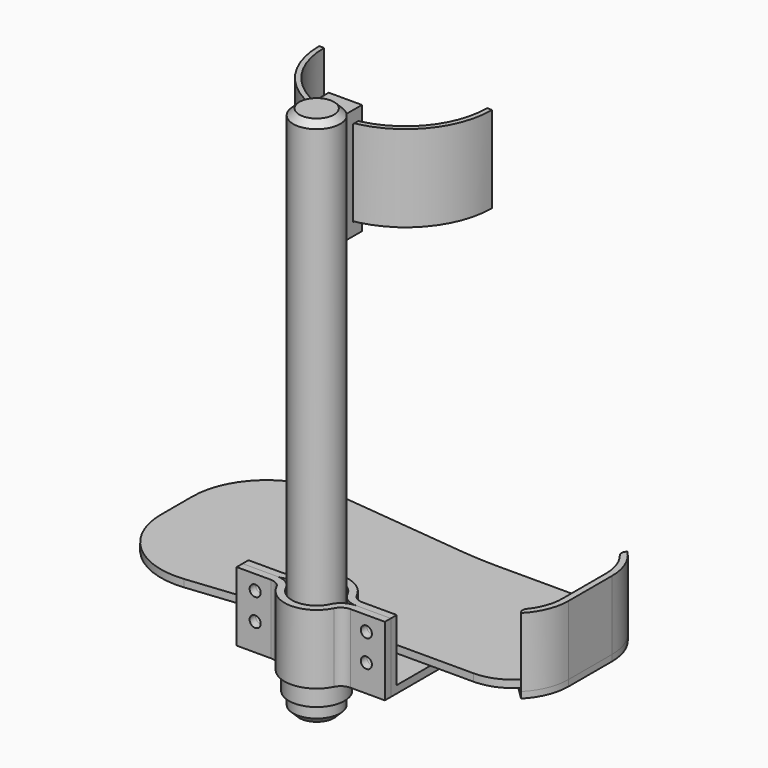
from build123d import *

# Parameters (mm, degrees)
F1_DEPTH  = 6
F2_R      = 60
F3_R      = 40
F4_R      = 300
F5_R      = 10
F6_DEPTH  = 6
F8_DEPTH  = 6
F9_DEPTH  = 50
F10_R     = 5
F12_DEPTH = 5
F14_DEPTH = 6
F16_DEPTH = 50
F17_R     = 10
F18_R     = 15
F20_DEPTH = 56
F21_R     = 4.5
F22_DEPTH = 25
F23_R     = 4.5
F24_DEPTH = 25
F25_R     = 19
F26_DEPTH = 400
F27_DEPTH = 30
F28_SIZE  = 5
F29_R     = 22.5
F29_R_2   = 19
F30_DEPTH = 15
F31_SIZE  = 5
F34_DEPTH = 90
F36_W     = 26.8700576851
F36_H     = 4
F37_DEPTH = 70
F39_DEPTH = 70


with BuildPart() as f1:
    # F0 (on Top) → F1 (new body)
    with BuildSketch(Plane.XY):
        Polygon((20, 62.0046741232), (-175, 82.5), (-175, -82.5), (20, -62.0046741232), (155, -62.0046741232), (155, 62.0046741232), align=None)
    extrude(amount=F1_DEPTH)

    # F2
    f2_edges = [f1.edges().sort_by_distance(p)[0] for p in [
        (-175, -82.5, 3),
        (-175, 82.5, 3),
    ]]
    fillet(f2_edges, radius=F2_R)

    # F3
    f3_edges = [f1.edges().sort_by_distance(p)[0] for p in [
        (155, 62.004674, 3),
        (155, -62.004674, 3),
    ]]
    fillet(f3_edges, radius=F3_R)

    # F4
    f4_edges = [f1.edges().sort_by_distance(p)[0] for p in [
        (20, -62.004674, 3),
        (20, 62.004674, 3),
    ]]
    fillet(f4_edges, radius=F4_R)

    # F5 (on Front) → F6 (join, symmetric)
    with BuildSketch(Plane.XZ):
        with BuildLine():
            Line((-30, 0), (5.2477547929, -38.5044904143))
            ThreePointArc((5.2477547929, -38.5044904143), (20, -45), (34.7522452071, -38.5044904143))
            Line((34.7522452071, -38.5044904143), (70, 0))
            Line((70, 0), (-30, 0))
        make_face()
        with Locations((20, -25)):
            Circle(F5_R, mode=Mode.SUBTRACT)
    extrude(amount=F6_DEPTH, both=True)

    # F23 (on face) → F24 (cut)
    with BuildSketch(Plane(origin=(0, -96.0046741232, 0), x_dir=(-1, 0, 0), z_dir=(0, 1, 0))):
        with Locations((25, 38)):
            Circle(F23_R)
        with Locations((25, 16)):
            Circle(F23_R)
        with Locations((-65, 38)):
            Circle(F23_R)
        with Locations((-65, 16)):
            Circle(F23_R)
    extrude(amount=-F24_DEPTH, mode=Mode.SUBTRACT)


with BuildPart() as f8:
    # F7 (on face) → F8 (new body)
    with BuildSketch(Plane.XY.offset(6)):
        with BuildLine():
            ThreePointArc((143.2842712475, 50.2889453707), (151.9551813005, 37.3120114178), (155, 22.0046741232))
            Line((155, 22.0046741232), (155, -22.0046741232))
            ThreePointArc((155, -22.0046741232), (151.9551813005, -37.3120114178), (143.2842712475, -50.2889453707))
            Line((143.2842712475, -50.2889453707), (146.8198051534, -53.8244792766))
            ThreePointArc((146.8198051534, -53.8244792766), (156.574578963, -39.2254285796), (160, -22.0046741232))
            Line((160, -22.0046741232), (160, 22.0046741232))
            ThreePointArc((160, 22.0046741232), (156.574578963, 39.2254285796), (146.8198051534, 53.8244792766))
            Line((146.8198051534, 53.8244792766), (143.2842712475, 50.2889453707))
        make_face()
    extrude(amount=-F8_DEPTH)

    # F7 (on face) → F9 (join)
    with BuildSketch(Plane.XY.offset(6)):
        with BuildLine():
            ThreePointArc((143.2842712475, 50.2889453707), (151.9551813005, 37.3120114178), (155, 22.0046741232))
            Line((155, 22.0046741232), (155, -22.0046741232))
            ThreePointArc((155, -22.0046741232), (151.9551813005, -37.3120114178), (143.2842712475, -50.2889453707))
            Line((143.2842712475, -50.2889453707), (146.8198051534, -53.8244792766))
            ThreePointArc((146.8198051534, -53.8244792766), (156.574578963, -39.2254285796), (160, -22.0046741232))
            Line((160, -22.0046741232), (160, 22.0046741232))
            ThreePointArc((160, 22.0046741232), (156.574578963, 39.2254285796), (146.8198051534, 53.8244792766))
            Line((146.8198051534, 53.8244792766), (143.2842712475, 50.2889453707))
        make_face()
    extrude(amount=F9_DEPTH)

    # F10
    f10_edges = [f8.edges().sort_by_distance(p)[0] for p in [
        (143.284271, -50.288945, 28),
        (143.284271, 50.288945, 28),
    ]]
    fillet(f10_edges, radius=F10_R)


with BuildPart() as f12:
    # F11 (on face) → F12 (new body)
    with BuildSketch(Plane(origin=(0, 0, 0), x_dir=(1, 0, 0), z_dir=(0, 0, -1))):
        with BuildLine():
            ThreePointArc((160, 22.0046741232), (156.574578963, 39.2254285796), (146.8198051534, 53.8244792766))
            Line((146.8198051534, 53.8244792766), (115, 22.0046741232))
            Line((115, 22.0046741232), (115, -22.0046741232))
            Line((115, -22.0046741232), (146.8198051534, -53.8244792766))
            ThreePointArc((146.8198051534, -53.8244792766), (156.574578963, -39.2254285796), (160, -22.0046741232))
            Line((160, -22.0046741232), (160, 22.0046741232))
        make_face()
    extrude(amount=F12_DEPTH)


with BuildPart() as f14:
    # F13 (on face) → F14 (new body)
    with BuildSketch(Plane(origin=(0, 0, 0), x_dir=(1, 0, 0), z_dir=(0, 0, -1))):
        with BuildLine():
            Line((0, 102.0046741232), (-40, 102.0046741232))
            Line((-40, 102.0046741232), (-40, 68.3109282391))
            Line((-40, 68.3109282391), (4.3637948046, 63.6481055127))
            ThreePointArc((4.3637948046, 63.6481055127), (20.021546912, 62.4158136968), (35.7223337849, 62.0046741232))
            Line((35.7223337849, 62.0046741232), (80, 62.0046741232))
            Line((80, 62.0046741232), (80, 102.0046741232))
            Line((80, 102.0046741232), (40, 102.0046741232))
            ThreePointArc((40, 102.0046741232), (20, 82.0046741232), (0, 102.0046741232))
        make_face()
        with BuildLine():
            Line((4.3637948046, 63.6481055127), (-40, 68.3109282391))
            Line((-40, 68.3109282391), (-40, 32.0046741232))
            Line((-40, 32.0046741232), (80, 32.0046741232))
            Line((80, 32.0046741232), (80, 62.0046741232))
            Line((80, 62.0046741232), (35.7223337849, 62.0046741232))
            ThreePointArc((35.7223337849, 62.0046741232), (20.021546912, 62.4158136968), (4.3637948046, 63.6481055127))
        make_face()
    extrude(amount=F14_DEPTH)

    # F15 (on face) → F16 (join)
    with BuildSketch(Plane.XY):
        with BuildLine():
            Line((-40, -102.0046741232), (0, -102.0046741232))
            ThreePointArc((0, -102.0046741232), (20, -82.0046741232), (40, -102.0046741232))
            Line((40, -102.0046741232), (80, -102.0046741232))
            Line((80, -102.0046741232), (80, -96.0046741232))
            Line((80, -96.0046741232), (45.2982212813, -96.0046741232))
            ThreePointArc((45.2982212813, -96.0046741232), (20, -76.0046741232), (-5.2982212813, -96.0046741232))
            Line((-5.2982212813, -96.0046741232), (-40, -96.0046741232))
            Line((-40, -96.0046741232), (-40, -102.0046741232))
        make_face()
    extrude(amount=F16_DEPTH)

    # F17
    f17_edges = [f14.edges().sort_by_distance(p)[0] for p in [
        (-5.298221, -96.004674, 25),
        (45.298221, -96.004674, 25),
    ]]
    fillet(f17_edges, radius=F17_R)

    # F18
    f18_edges = [f14.edges().sort_by_distance(p)[0] for p in [
        (40, -102.004674, 22),
        (0, -102.004674, 22),
    ]]
    fillet(f18_edges, radius=F18_R)


with BuildPart() as f20:
    # F19 (on face) → F20 (new body)
    with BuildSketch(Plane.XY.offset(50)):
        with BuildLine():
            Line((-11.6227766017, -102.0046741232), (-40, -102.0046741232))
            Line((-40, -102.0046741232), (-40, -108.0046741232))
            Line((-40, -108.0046741232), (-12.2490309932, -108.0046741232))
            ThreePointArc((-12.2490309932, -108.0046741232), (-6.9785682262, -109.5063082672), (-3.2909668284, -113.5602296787))
            ThreePointArc((-3.2909668284, -113.5602296787), (20, -128.0046741232), (43.2909668284, -113.5602296787))
            ThreePointArc((43.2909668284, -113.5602296787), (46.9785682262, -109.5063082672), (52.2490309932, -108.0046741232))
            Line((52.2490309932, -108.0046741232), (80, -108.0046741232))
            Line((80, -108.0046741232), (80, -102.0046741232))
            Line((80, -102.0046741232), (51.6227766017, -102.0046741232))
            ThreePointArc((51.6227766017, -102.0046741232), (43.6049393443, -104.3273603023), (38.0701580581, -110.5761026946))
            ThreePointArc((38.0701580581, -110.5761026946), (20, -122.0046741232), (1.9298419419, -110.5761026946))
            ThreePointArc((1.9298419419, -110.5761026946), (-3.6049393443, -104.3273603023), (-11.6227766017, -102.0046741232))
        make_face()
    extrude(amount=-F20_DEPTH)


with BuildPart() as f22_tool:
    # F21 (on face) → F22 (new body)
    with BuildSketch(Plane.XZ.offset(108.0046741232)):
        with Locations((-25, 38)):
            Circle(F21_R)
        with Locations((-25, 16)):
            Circle(F21_R)
        with Locations((65, 38)):
            Circle(F21_R)
        with Locations((65, 16)):
            Circle(F21_R)
    extrude(amount=-F22_DEPTH)


with BuildPart() as f14_1:
    add(f14.part)

    # F22: cut by f22_tool
    add(f22_tool.part, mode=Mode.SUBTRACT)


with BuildPart() as f20_1:
    add(f20.part)

    # F22: cut by f22_tool
    add(f22_tool.part, mode=Mode.SUBTRACT)


with BuildPart() as f26:
    # F25 (on face) → F26 (new body)
    with BuildSketch(Plane(origin=(0, 0, -6), x_dir=(1, 0, 0), z_dir=(0, 0, -1))):
        with Locations((20, 102.0046741232)):
            Circle(F25_R)
    extrude(amount=-F26_DEPTH)

    # F27 (add): a face of the model
    f27_faces = [f26.faces().sort_by_distance(p)[0] for p in [
        (20, -102.0046741232, -6),
    ]]
    extrude(f27_faces, amount=F27_DEPTH)

    # F28
    f28_edges = [f26.edges().sort_by_distance(p)[0] for p in [
        (1, -102.004674, -36),
    ]]
    chamfer(f28_edges, length=F28_SIZE)

    # F31
    f31_edges = [f26.edges().sort_by_distance(p)[0] for p in [
        (1, -102.004674, 394),
    ]]
    chamfer(f31_edges, length=F31_SIZE)


with BuildPart() as f30:
    # F29 (on face) → F30 (new body)
    with BuildSketch(Plane(origin=(0, 0, -6), x_dir=(1, 0, 0), z_dir=(0, 0, -1))):
        with Locations((20, 102.0046741232)):
            Circle(F29_R)
        with Locations((20, 102.0046741232)):
            Circle(F29_R_2, mode=Mode.SUBTRACT)
    extrude(amount=F30_DEPTH)


with BuildPart() as f34:
    # F33 (on offset) → F34 (new body)
    with BuildSketch(Plane.XY.offset(389)):
        with BuildLine():
            Line((33.4350288425, -88.5696452806), (33.4350288425, -73.0046741232))
            Line((33.4350288425, -73.0046741232), (6.5649711575, -73.0046741232))
            Line((6.5649711575, -73.0046741232), (6.5649711575, -88.5696452806))
            ThreePointArc((6.5649711575, -88.5696452806), (20, -83.0046741232), (33.4350288425, -88.5696452806))
        make_face()
    extrude(amount=-F34_DEPTH)

    # F36 (on offset) → F37 (cut)
    with BuildSketch(Plane.XY.offset(379)):
        with Locations((20, -80.0046741232)):
            Rectangle(F36_W, F36_H)
    extrude(amount=-F37_DEPTH, mode=Mode.SUBTRACT)


with BuildPart() as f39:
    # F38 (on offset) → F39 (new body)
    with BuildSketch(Plane.XY.offset(379)):
        with BuildLine():
            Line((-46, -12.0046741232), (-50, -12.0046741232))
            ThreePointArc((-50, -12.0046741232), (-29.4974746831, -61.5021488063), (20, -82.0046741232))
            ThreePointArc((20, -82.0046741232), (69.4974746831, -61.5021488063), (90, -12.0046741232))
            Line((90, -12.0046741232), (86, -12.0046741232))
            ThreePointArc((86, -12.0046741232), (20, -78.0046741232), (-46, -12.0046741232))
        make_face()
    extrude(amount=-F39_DEPTH)


solid = Compound([f1.part, f8.part, f12.part, f14_1.part, f20_1.part, f26.part, f30.part, f34.part, f39.part])
